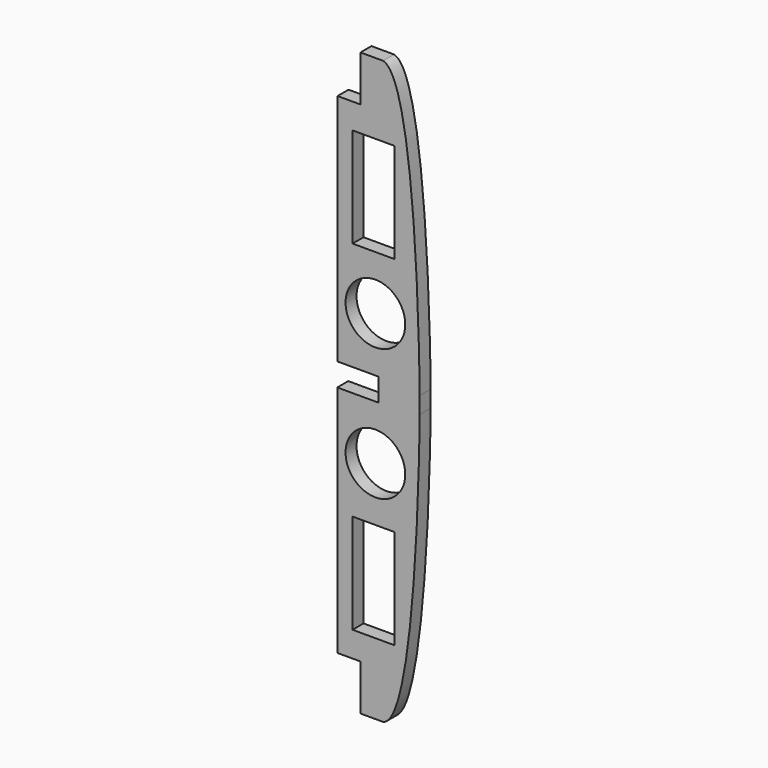
from build123d import *

# Parameters (mm, degrees)
F0_R     = 13.033720186
F0_W     = 18.248938024
F0_H     = 43.4933193028
F1_DEPTH = 6


# Not quite as in the source:
# - a feature names something its author has since deleted; it is built from what else it names


with BuildPart() as f1:
    # F0 (on Front) → F1 (new body)
    with BuildSketch(Plane.XZ):
        with BuildLine():
            add(Edge.make_bspline(
                [(105.1375677345, 103.5958733921), (118.915635106, 100.3235823913), (120.9318600426, 1.7429371205), (121.1375677345, -19.7457277863)],
                knots=[0, 0, 0, 0, 110.2279027072, 110.2279027072, 110.2279027072, 110.2279027072], degree=3))
            Line((105.1375677345, 103.5958733921), (95.2585982296, 103.5958733921))
            Line((95.2585982296, 103.5958733921), (95.2585982296, 83.5958733921))
            Line((95.2585982296, 83.5958733921), (85.2585982296, 83.5958733921))
            Line((85.2585982296, 83.5958733921), (85.2585982296, 62.4470586631))
            Line((85.2585982296, 62.4470586631), (85.1375677345, -18.4041266079))
            Line((85.1375677345, -18.4041266079), (103.1375677345, -18.4041266079))
            Line((103.1375677345, -18.4041266079), (103.1375677345, -23.4041266079))
            Line((103.1375677345, -23.4041266079), (121.1375677345, -23.4041266079))
            Line((121.1375677345, -23.4041266079), (121.1375677345, -19.7457277863))
        make_face()
        with Locations((101.7788599941, 5.3969110339)):
            Circle(F0_R, mode=Mode.SUBTRACT)
        with Locations((100.9382642806, 50.7787894458)):
            Rectangle(F0_W, F0_H, mode=Mode.SUBTRACT)
        with BuildLine():
            Line((121.1375677345, -27.0625254295), (121.1375677345, -23.4041266079))
            Line((121.1375677345, -23.4041266079), (103.1375677345, -23.4041266079))
            Line((103.1375677345, -23.4041266079), (103.1375677345, -28.4041266079))
            Line((103.1375677345, -28.4041266079), (85.1375677345, -28.4041266079))
            Line((85.1375677345, -28.4041266079), (85.2585982296, -130.4041266079))
            Line((85.2585982296, -130.4041266079), (95.2585982296, -130.4041266079))
            Line((95.2585982296, -130.4041266079), (95.2585982296, -150.4041266079))
            Line((95.2585982296, -150.4041266079), (105.1375677345, -150.4041266079))
            add(Edge.make_bspline(
                [(105.1375677345, -150.4041266079), (118.915635106, -147.1318356072), (120.9318600426, -48.5511903363), (121.1375677345, -27.0625254295)],
                knots=[0, 0, 0, 0, 110.2279027072, 110.2279027072, 110.2279027072, 110.2279027072], degree=3))
        make_face()
        with Locations((100.9382642806, -97.5870426616)):
            Rectangle(F0_W, F0_H, mode=Mode.SUBTRACT)
        with Locations((101.7788599941, -52.2051642497)):
            Circle(F0_R, mode=Mode.SUBTRACT)
    extrude(amount=F1_DEPTH)


solid = f1.part
